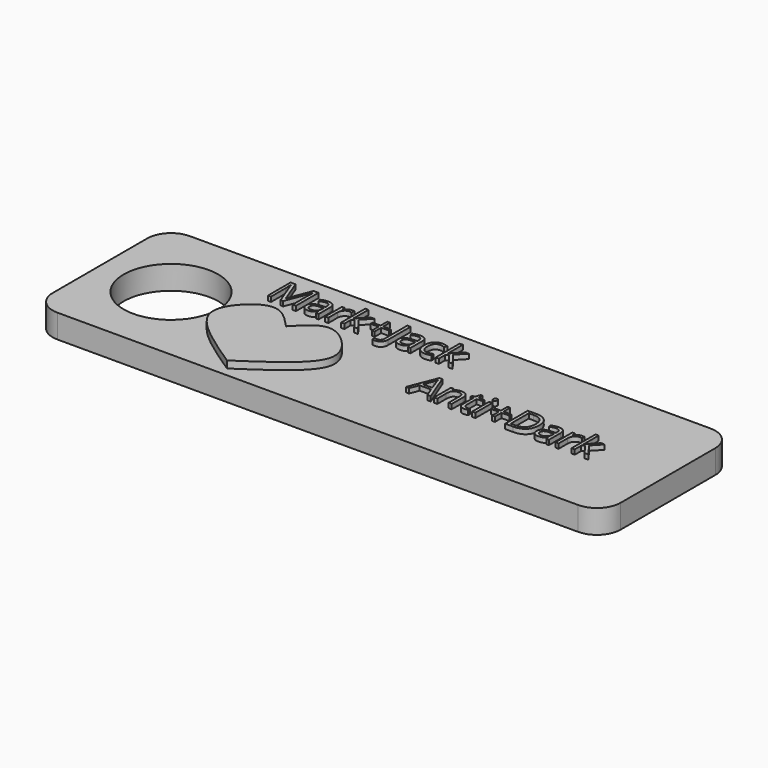
from build123d import *

# Parameters (mm, degrees)
F0_W         = 120
F0_H         = 35
F0_R         = 10
F1_DEPTH     = 5
F2_R         = 5
F3_R         = 5
F4_R         = 5
F5_R         = 5
F6_TEXT_SIZE = 8.3333333333
F7_DEPTH     = 6
F9_DEPTH     = 1.5


# Not quite as in the source:
# - Text() gives the source's letters only with a copy of the font that has no kerning and outlines rounded to 1/6400 em; it was checked with that copy


with BuildPart() as f1:
    # F0 (on Top) → F1 (new body)
    with BuildSketch(Plane.XY):
        Rectangle(F0_W, F0_H)
        with Locations((-45, 0)):
            Circle(F0_R, mode=Mode.SUBTRACT)
    extrude(amount=F1_DEPTH)

    # F2
    f2_edges = [f1.edges().sort_by_distance(p)[0] for p in [
        (60, -17.5, 2.5),
    ]]
    fillet(f2_edges, radius=F2_R)

    # F3
    f3_edges = [f1.edges().sort_by_distance(p)[0] for p in [
        (60, 17.5, 2.5),
    ]]
    fillet(f3_edges, radius=F3_R)

    # F4
    f4_edges = [f1.edges().sort_by_distance(p)[0] for p in [
        (-60, 17.5, 2.5),
    ]]
    fillet(f4_edges, radius=F4_R)

    # F5
    f5_edges = [f1.edges().sort_by_distance(p)[0] for p in [
        (-60, -17.5, 2.5),
    ]]
    fillet(f5_edges, radius=F5_R)

    # F6 (on Top) → F7 (join)
    with BuildSketch(Plane.XY):
        with Locations((-31.3137767383, 7.4999993836)):
            Text('Mark+Jack', F6_TEXT_SIZE, font='Open Sans', text_align=(TextAlign.LEFT, TextAlign.BOTTOM))
        with Locations((7.6627857617, -3.8333339498)):
            Text('Anti+Dark', F6_TEXT_SIZE, font='Open Sans', text_align=(TextAlign.LEFT, TextAlign.BOTTOM))
    extrude(amount=F7_DEPTH)

    # F8 (on face) → F9 (join)
    with BuildSketch(Plane.XY.offset(5)):
        with BuildLine():
            add(Edge.make_bspline(
                [(-20.6925105304, 0), (-18.8244686793, 2.0127007773), (-15.0883847756, 6.038102549), (-8.1879868901, 0.257971721), (-6.8682594334, -6.4391965409), (-15.324783633, -12.0471754478), (-20.6925105304, -15.6068056822)],
                knots=[0, 0, 0, 0, 0.2289956362, 0.457991297, 0.6559632983, 1, 1, 1, 1], degree=3))
            add(Edge.make_bspline(
                [(-20.6925105304, 0), (-22.5605523814, 2.0127007773), (-26.2966362851, 6.038102549), (-33.1970341706, 0.257971721), (-34.5167616273, -6.4391965409), (-26.0602374277, -12.0471754478), (-20.6925105304, -15.6068056822)],
                knots=[0, 0, 0, 0, 0.2289956362, 0.457991297, 0.6559632983, 1, 1, 1, 1], degree=3))
        make_face()
    extrude(amount=F9_DEPTH)


solid = f1.part
